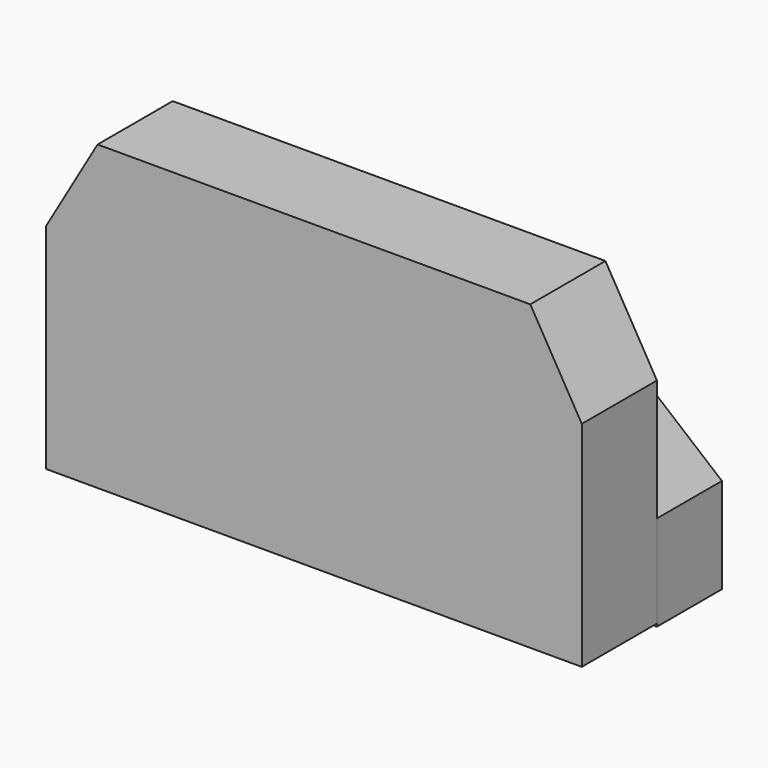
from build123d import *

# Parameters (mm, degrees)
F1_DEPTH    = 17.018
F3_DEPTH    = 17.272
F4_W        = 11.0760657117
F4_H        = 15.8854108304
F4_W_2      = 11.9504909962
F5_DEPTH    = 19.812
F6_T4_DEPTH = 141.7175615003


# Not quite as in the source:
# - a fillet or chamfer that OpenCascade refuses, or shapes differently, is made with other operations: its cross-section is extruded or revolved along the edge and cut away or added
# - a feature of the source that left no trace in its solid (it failed there, or was rolled back) is left out


with BuildPart() as f1:
    # F0 (on Front) → F1 (new body)
    with BuildSketch(Plane.XZ):
        Polygon((-58.5865564644, 22.0063943416), (-58.5865564644, -16.7598351836), (38.4747292797, -16.7598351836), (38.4747292797, 22.0063943416), (29.1475392878, 38.0375422537), (-49.2593459785, 38.0375422537), align=None)
    extrude(amount=F1_DEPTH)

    # F2 (on Top) → F3 (join)
    with BuildSketch(Plane.XY):
        Polygon((-58.5865564644, 14.7195085883), (-58.5865564644, 0), (38.4747572243, 0), (38.4747572243, 14.7195085883), (-2.6232791133, 40.3693430126), align=None)
    extrude(amount=-F3_DEPTH)

    # F4 (on face) → F5 (join)
    with BuildSketch(Plane(origin=(0, 0, 0), x_dir=(-1, 0, 0), z_dir=(0, 1, 0))):
        with Locations((-14.282295946, 7.9427054152)):
            Rectangle(F4_W, F4_H)
        with Locations((33.6654121056, 7.9427054152)):
            Rectangle(F4_W_2, F4_H)
    extrude(amount=F5_DEPTH)

    # F6: chamfer of 25.4 on 1 edges, made by hand


with BuildPart() as f6_tool2:
    # F6_s3 → F6_t4 (new body)
    with BuildSketch(Plane.YZ.offset(-56.5764848041)):
        Polygon((19.812, -9.5145891696), (-5.588, 15.8854108304), (19.812, 15.8854108304), align=None)
    extrude(amount=F6_T4_DEPTH)

    split(bisect_by=Plane.XY, keep=Keep.TOP)

    split(bisect_by=Plane.XZ, keep=Keep.BOTTOM)


with BuildPart() as f1_1:
    add(f1.part)

    # F6_t1: cut F6_tool2
    add(f6_tool2.part, mode=Mode.SUBTRACT)


solid = f1_1.part
